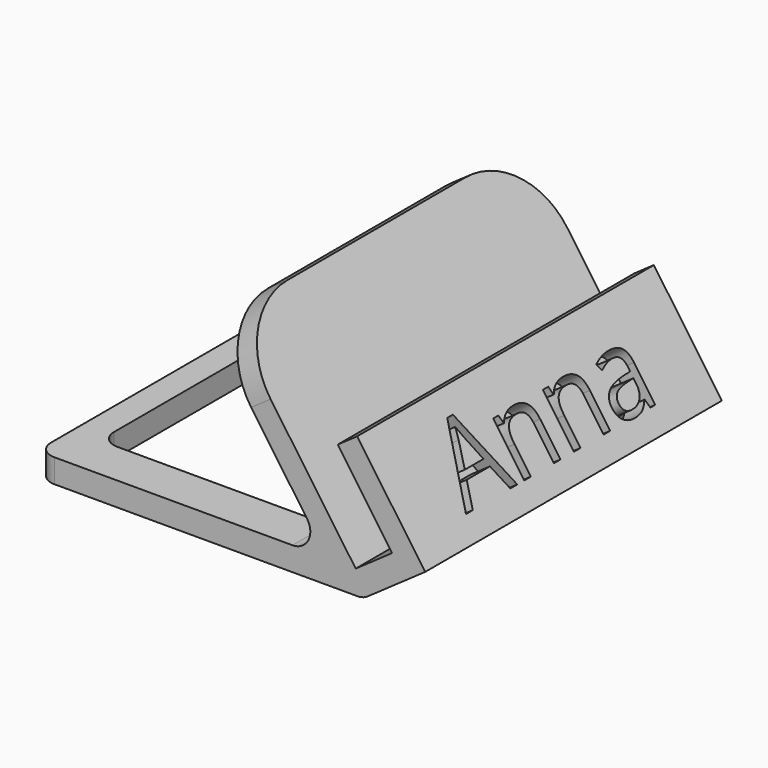
from build123d import *

# Parameters (mm, degrees)
F1_DEPTH     = 25
F4_W         = 14.7076435969
F4_H         = 20.1878626859
F5_DEPTH     = 25
F6_R         = 1.2
F7_R         = 5
F8_TEXT_SIZE = 6.8277055915
F9_DEPTH     = 2


# Not quite as in the source:
# - a feature of the source that left no trace in its solid (it failed there, or was rolled back) is left out
# - Text() gives the source's letters only with a copy of the font that has no kerning and outlines rounded to 1/6400 em; it was checked with that copy


with BuildPart() as f1:
    # F0 (on Front) → F1 (new body)
    with BuildSketch(Plane.XZ):
        Polygon((0, 1.6), (0, 0), (22, 0), (26.1813436397, 2.9278083364), (21.5927321489, 9.4810246907), (20.282088878, 8.5633023925), (23.9529780707, 3.3207293091), (21.4955219378, 1.6), (12.8918753925, 13.8872806643), (11.5812321217, 12.9695583662), (19.5422825958, 1.6), align=None)
    extrude(amount=F1_DEPTH)

    # F4 (on face) → F5 (cut)
    with BuildSketch(Plane.XY.offset(1.6)):
        with Locations((9.1884607973, -11.9060686571)):
            Rectangle(F4_W, F4_H)
    extrude(amount=-F5_DEPTH, mode=Mode.SUBTRACT)

    # F6
    f6_edges = [f1.edges().sort_by_distance(p)[0] for p in [
        (22, -12.5, 0),
        (0, -25, 0.8),
        (1.834639, -22, 0.8),
        (1.834639, -1.812137, 0.8),
        (0, 0, 0.8),
        (19.542283, -12.5, 1.6),
    ]]
    fillet(f6_edges, radius=F6_R)

    # F7
    f7_edges = [f1.edges().sort_by_distance(p)[0] for p in [
        (12.236554, -25, 13.42842),
        (12.236554, 0, 13.42842),
    ]]
    fillet(f7_edges, radius=F7_R)

    # F8 (on face) → F9 (cut)
    with BuildSketch(Plane(origin=(18.9435652163, 0, 13.264427165), x_dir=(0, 1, 0), z_dir=(0.8191520443, 0, 0.5735764364))):
        with Locations((-20.4380722716, -11.0491761006)):
            Text('Anna', F8_TEXT_SIZE, font='Open Sans', text_align=(TextAlign.LEFT, TextAlign.BOTTOM))
    extrude(amount=-F9_DEPTH, mode=Mode.SUBTRACT)


solid = f1.part
